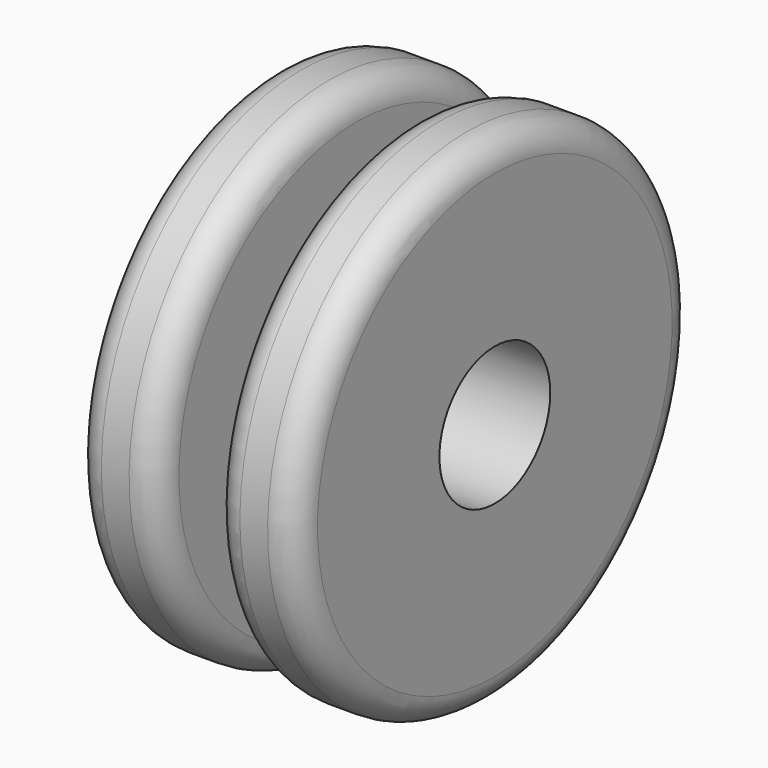
from build123d import *

# Parameters (mm, degrees)
F2_R     = 3.175
F3_DEPTH = 25.4
F4_R     = 1.26999


# Not quite as in the source:
# - a fillet or chamfer is up to 0.001 mm smaller than in the source, because OpenCascade refuses the exact size


with BuildPart() as f1:
    # F0 (on Front) → F1 (revolve)
    with BuildSketch(Plane.XZ):
        Polygon((0, 11.43), (0, 0), (10.16, 0), (10.16, 11.43), (6.35, 11.43), (6.35, 5.08), (3.81, 5.08), (3.81, 11.43), align=None)
    revolve(axis=Axis((5.08, 0, 0), (1, 0, 0)))

    # F2 (on face) → F3 (cut)
    with BuildSketch(Plane.YZ.offset(10.16)):
        Circle(F2_R)
    extrude(amount=-F3_DEPTH, mode=Mode.SUBTRACT)

    # F4 (radius 1.27 in the source; OpenCascade refuses exactly that, so slightly less here)
    f4_edges = [f1.edges().sort_by_distance(p)[0] for p in [
        (6.35, 0, -5.08),
        (3.81, 0, -5.08),
        (3.81, 0, -11.43),
        (0, 0, -11.43),
        (10.16, 0, -11.43),
        (6.35, 0, -11.43),
    ]]
    fillet(f4_edges, radius=F4_R)


solid = f1.part
